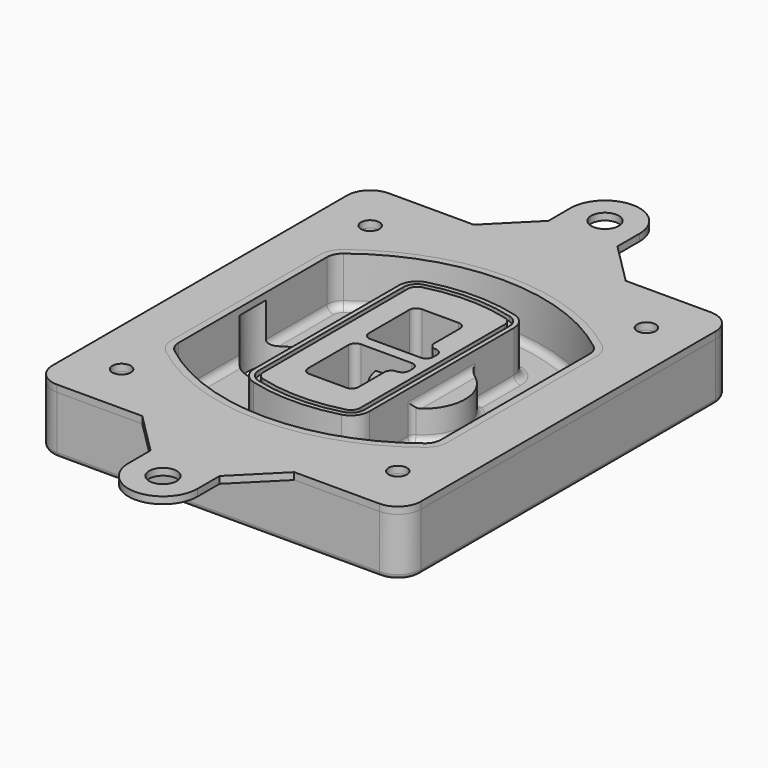
from build123d import *

# Parameters (mm, degrees)
F0_R      = 4
F1_DEPTH  = 25
F2_DEPTH  = 3
F3_DEPTH  = 18
F5_DEPTH  = 21
F6_DEPTH  = 2
F8_DEPTH  = 20
F9_DEPTH  = 16
F10_DEPTH = 25
F7_R      = 6
F7_R_2    = 4
F11_DEPTH = 6
F13_DEPTH = 9
F14_R     = 3
F15_R     = 2
F16_R     = 6
F16_R_2   = 4
F17_DEPTH = 3


# Not quite as in the source:
# - a feature names something its author has since deleted; it is built from what else it names


with BuildPart() as f1:
    # F0 (on Top) → F1 (new body)
    with BuildSketch(Plane.XY):
        with BuildLine():
            ThreePointArc((-80, -80), (-77.0710678119, -87.0710678119), (-70, -90))
            Line((-70, -90), (70, -90))
            ThreePointArc((70, -90), (77.0710678119, -87.0710678119), (80, -80))
            Line((80, -80), (80, 80))
            ThreePointArc((80, 80), (77.0710678119, 87.0710678119), (70, 90))
            Line((70, 90), (-70, 90))
            ThreePointArc((-70, 90), (-77.0710678119, 87.0710678119), (-80, 80))
            Line((-80, 80), (-80, -80))
        make_face()
        with Locations((-60, -67.5)):
            Circle(F0_R, mode=Mode.SUBTRACT)
        with Locations((60, -67.5)):
            Circle(F0_R, mode=Mode.SUBTRACT)
        with Locations((-60, 67.5)):
            Circle(F0_R, mode=Mode.SUBTRACT)
        with BuildLine():
            ThreePointArc((-64, 40.2934422872), (-62.5820384798, 46.4328484224), (-58.6153846154, 51.3286200352))
            ThreePointArc((-58.6153846154, 51.3286200352), (0, 71.5), (58.6153846154, 51.3286200352))
            ThreePointArc((58.6153846154, 51.3286200352), (62.5820384798, 46.4328484224), (64, 40.2934422872))
            Line((64, 40.2934422872), (64, -40.2934422872))
            ThreePointArc((64, -40.2934422872), (62.5820384798, -46.4328484224), (58.6153846154, -51.3286200352))
            ThreePointArc((58.6153846154, -51.3286200352), (0, -71.5), (-58.6153846154, -51.3286200352))
            ThreePointArc((-58.6153846154, -51.3286200352), (-62.5820384798, -46.4328484224), (-64, -40.2934422872))
            Line((-64, -40.2934422872), (-64, 40.2934422872))
        make_face(mode=Mode.SUBTRACT)
        with Locations((60, 67.5)):
            Circle(F0_R, mode=Mode.SUBTRACT)
        with BuildLine():
            ThreePointArc((58.6153846154, 51.3286200352), (0, 71.5), (-58.6153846154, 51.3286200352))
            ThreePointArc((-58.6153846154, 51.3286200352), (-62.5820384798, 46.4328484224), (-64, 40.2934422872))
            Line((-64, 40.2934422872), (-64, -40.2934422872))
            ThreePointArc((-64, -40.2934422872), (-62.5820384798, -46.4328484224), (-58.6153846154, -51.3286200352))
            ThreePointArc((-58.6153846154, -51.3286200352), (0, -71.5), (58.6153846154, -51.3286200352))
            ThreePointArc((58.6153846154, -51.3286200352), (62.5820384798, -46.4328484224), (64, -40.2934422872))
            Line((64, -40.2934422872), (64, 40.2934422872))
            ThreePointArc((64, 40.2934422872), (62.5820384798, 46.4328484224), (58.6153846154, 51.3286200352))
        make_face()
        with BuildLine():
            Line((-60, -40.2934422872), (-60, 40.2934422872))
            ThreePointArc((-60, 40.2934422872), (-58.9871703427, 44.6787323838), (-56.1538461538, 48.1757121072))
            ThreePointArc((-56.1538461538, 48.1757121072), (0, 67.5), (56.1538461538, 48.1757121072))
            ThreePointArc((56.1538461538, 48.1757121072), (58.9871703427, 44.6787323838), (60, 40.2934422872))
            Line((60, 40.2934422872), (60, -40.2934422872))
            ThreePointArc((60, -40.2934422872), (58.9871703427, -44.6787323838), (56.1538461538, -48.1757121072))
            ThreePointArc((56.1538461538, -48.1757121072), (0, -67.5), (-56.1538461538, -48.1757121072))
            ThreePointArc((-56.1538461538, -48.1757121072), (-58.9871703427, -44.6787323838), (-60, -40.2934422872))
        make_face(mode=Mode.SUBTRACT)
        with BuildLine():
            ThreePointArc((-56.1538461538, 48.1757121072), (-58.9871703427, 44.6787323838), (-60, 40.2934422872))
            Line((-60, 40.2934422872), (-60, -40.2934422872))
            ThreePointArc((-60, -40.2934422872), (-58.9871703427, -44.6787323838), (-56.1538461538, -48.1757121072))
            ThreePointArc((-56.1538461538, -48.1757121072), (0, -67.5), (56.1538461538, -48.1757121072))
            ThreePointArc((56.1538461538, -48.1757121072), (58.9871703427, -44.6787323838), (60, -40.2934422872))
            Line((60, -40.2934422872), (60, 40.2934422872))
            ThreePointArc((60, 40.2934422872), (58.9871703427, 44.6787323838), (56.1538461538, 48.1757121072))
            ThreePointArc((56.1538461538, 48.1757121072), (0, 67.5), (-56.1538461538, 48.1757121072))
        make_face()
        with BuildLine():
            ThreePointArc((54.3076923077, 45.8110311612), (56.2910192399, 43.3631453548), (57, 40.2934422872))
            Line((57, 40.2934422872), (57, -40.2934422872))
            ThreePointArc((57, -40.2934422872), (56.2910192399, -43.3631453548), (54.3076923077, -45.8110311612))
            ThreePointArc((54.3076923077, -45.8110311612), (0, -64.5), (-54.3076923077, -45.8110311612))
            ThreePointArc((-54.3076923077, -45.8110311612), (-56.2910192399, -43.3631453548), (-57, -40.2934422872))
            Line((-57, -40.2934422872), (-57, 40.2934422872))
            ThreePointArc((-57, 40.2934422872), (-56.2910192399, 43.3631453548), (-54.3076923077, 45.8110311612))
            ThreePointArc((-54.3076923077, 45.8110311612), (0, 64.5), (54.3076923077, 45.8110311612))
        make_face(mode=Mode.SUBTRACT)
        with BuildLine():
            Line((57, -40.2934422872), (57, 40.2934422872))
            ThreePointArc((57, 40.2934422872), (56.2910192399, 43.3631453548), (54.3076923077, 45.8110311612))
            ThreePointArc((54.3076923077, 45.8110311612), (0, 64.5), (-54.3076923077, 45.8110311612))
            ThreePointArc((-54.3076923077, 45.8110311612), (-56.2910192399, 43.3631453548), (-57, 40.2934422872))
            Line((-57, 40.2934422872), (-57, -40.2934422872))
            ThreePointArc((-57, -40.2934422872), (-56.2910192399, -43.3631453548), (-54.3076923077, -45.8110311612))
            ThreePointArc((-54.3076923077, -45.8110311612), (0, -64.5), (54.3076923077, -45.8110311612))
            ThreePointArc((54.3076923077, -45.8110311612), (56.2910192399, -43.3631453548), (57, -40.2934422872))
        make_face()
    extrude(amount=-F1_DEPTH)

    # F0 (on Top) → F2 (join)
    with BuildSketch(Plane.XY):
        with BuildLine():
            ThreePointArc((-56.1538461538, 48.1757121072), (-58.9871703427, 44.6787323838), (-60, 40.2934422872))
            Line((-60, 40.2934422872), (-60, -40.2934422872))
            ThreePointArc((-60, -40.2934422872), (-58.9871703427, -44.6787323838), (-56.1538461538, -48.1757121072))
            ThreePointArc((-56.1538461538, -48.1757121072), (0, -67.5), (56.1538461538, -48.1757121072))
            ThreePointArc((56.1538461538, -48.1757121072), (58.9871703427, -44.6787323838), (60, -40.2934422872))
            Line((60, -40.2934422872), (60, 40.2934422872))
            ThreePointArc((60, 40.2934422872), (58.9871703427, 44.6787323838), (56.1538461538, 48.1757121072))
            ThreePointArc((56.1538461538, 48.1757121072), (0, 67.5), (-56.1538461538, 48.1757121072))
        make_face()
        with BuildLine():
            ThreePointArc((54.3076923077, 45.8110311612), (56.2910192399, 43.3631453548), (57, 40.2934422872))
            Line((57, 40.2934422872), (57, -40.2934422872))
            ThreePointArc((57, -40.2934422872), (56.2910192399, -43.3631453548), (54.3076923077, -45.8110311612))
            ThreePointArc((54.3076923077, -45.8110311612), (0, -64.5), (-54.3076923077, -45.8110311612))
            ThreePointArc((-54.3076923077, -45.8110311612), (-56.2910192399, -43.3631453548), (-57, -40.2934422872))
            Line((-57, -40.2934422872), (-57, 40.2934422872))
            ThreePointArc((-57, 40.2934422872), (-56.2910192399, 43.3631453548), (-54.3076923077, 45.8110311612))
            ThreePointArc((-54.3076923077, 45.8110311612), (0, 64.5), (54.3076923077, 45.8110311612))
        make_face(mode=Mode.SUBTRACT)
    extrude(amount=F2_DEPTH)

    # F0 (on Top) → F3 (cut)
    with BuildSketch(Plane.XY):
        with BuildLine():
            Line((57, -40.2934422872), (57, 40.2934422872))
            ThreePointArc((57, 40.2934422872), (56.2910192399, 43.3631453548), (54.3076923077, 45.8110311612))
            ThreePointArc((54.3076923077, 45.8110311612), (0, 64.5), (-54.3076923077, 45.8110311612))
            ThreePointArc((-54.3076923077, 45.8110311612), (-56.2910192399, 43.3631453548), (-57, 40.2934422872))
            Line((-57, 40.2934422872), (-57, -40.2934422872))
            ThreePointArc((-57, -40.2934422872), (-56.2910192399, -43.3631453548), (-54.3076923077, -45.8110311612))
            ThreePointArc((-54.3076923077, -45.8110311612), (0, -64.5), (54.3076923077, -45.8110311612))
            ThreePointArc((54.3076923077, -45.8110311612), (56.2910192399, -43.3631453548), (57, -40.2934422872))
        make_face()
    extrude(amount=-F3_DEPTH, mode=Mode.SUBTRACT)

    # F4 (on face) → F5 (join, through all)
    with BuildSketch(Plane.XY.offset(3)):
        with BuildLine():
            ThreePointArc((-25, -39.2465276821), (-23.3511545998, -44.1109737193), (-19.0842911877, -46.9702398883))
            ThreePointArc((-19.0842911877, -46.9702398883), (0, -49.5), (19.0842911877, -46.9702398883))
            ThreePointArc((19.0842911877, -46.9702398883), (23.3511545998, -44.1109737193), (25, -39.2465276821))
            Line((25, -39.2465276821), (25, 39.2465276821))
            ThreePointArc((25, 39.2465276821), (23.3511545998, 44.1109737193), (19.0842911877, 46.9702398883))
            ThreePointArc((19.0842911877, 46.9702398883), (0, 49.5), (-19.0842911877, 46.9702398883))
            ThreePointArc((-19.0842911877, 46.9702398883), (-23.3511545998, 44.1109737193), (-25, 39.2465276821))
            Line((-25, 39.2465276821), (-25, -39.2465276821))
        make_face()
        with BuildLine():
            ThreePointArc((18.5632183908, 45.0393118368), (21.7633659499, 42.89486221), (23, 39.2465276821))
            Line((23, 39.2465276821), (23, -39.2465276821))
            ThreePointArc((23, -39.2465276821), (21.7633659499, -42.89486221), (18.5632183908, -45.0393118368))
            ThreePointArc((18.5632183908, -45.0393118368), (0, -47.5), (-18.5632183908, -45.0393118368))
            ThreePointArc((-18.5632183908, -45.0393118368), (-21.7633659499, -42.89486221), (-23, -39.2465276821))
            Line((-23, -39.2465276821), (-23, 39.2465276821))
            ThreePointArc((-23, 39.2465276821), (-21.7633659499, 42.89486221), (-18.5632183908, 45.0393118368))
            ThreePointArc((-18.5632183908, 45.0393118368), (0, 47.5), (18.5632183908, 45.0393118368))
        make_face(mode=Mode.SUBTRACT)
        with BuildLine():
            Line((23, -39.2465276821), (23, 39.2465276821))
            ThreePointArc((23, 39.2465276821), (21.7633659499, 42.89486221), (18.5632183908, 45.0393118368))
            ThreePointArc((18.5632183908, 45.0393118368), (0, 47.5), (-18.5632183908, 45.0393118368))
            ThreePointArc((-18.5632183908, 45.0393118368), (-21.7633659499, 42.89486221), (-23, 39.2465276821))
            Line((-23, 39.2465276821), (-23, -39.2465276821))
            ThreePointArc((-23, -39.2465276821), (-21.7633659499, -42.89486221), (-18.5632183908, -45.0393118368))
            ThreePointArc((-18.5632183908, -45.0393118368), (0, -47.5), (18.5632183908, -45.0393118368))
            ThreePointArc((18.5632183908, -45.0393118368), (21.7633659499, -42.89486221), (23, -39.2465276821))
        make_face()
        with BuildLine():
            ThreePointArc((18.0421455939, 43.1083837852), (20.1755772999, 41.6787507007), (21, 39.2465276821))
            Line((21, 39.2465276821), (21, -39.2465276821))
            ThreePointArc((21, -39.2465276821), (20.1755772999, -41.6787507007), (18.0421455939, -43.1083837852))
            ThreePointArc((18.0421455939, -43.1083837852), (0, -45.5), (-18.0421455939, -43.1083837852))
            ThreePointArc((-18.0421455939, -43.1083837852), (-20.1755772999, -41.6787507007), (-21, -39.2465276821))
            Line((-21, -39.2465276821), (-21, 39.2465276821))
            ThreePointArc((-21, 39.2465276821), (-20.1755772999, 41.6787507007), (-18.0421455939, 43.1083837852))
            ThreePointArc((-18.0421455939, 43.1083837852), (0, 45.5), (18.0421455939, 43.1083837852))
        make_face(mode=Mode.SUBTRACT)
        with BuildLine():
            Line((21, -39.2465276821), (21, 39.2465276821))
            ThreePointArc((21, 39.2465276821), (20.1755772999, 41.6787507007), (18.0421455939, 43.1083837852))
            ThreePointArc((18.0421455939, 43.1083837852), (0, 45.5), (-18.0421455939, 43.1083837852))
            ThreePointArc((-18.0421455939, 43.1083837852), (-20.1755772999, 41.6787507007), (-21, 39.2465276821))
            Line((-21, 39.2465276821), (-21, -39.2465276821))
            ThreePointArc((-21, -39.2465276821), (-20.1755772999, -41.6787507007), (-18.0421455939, -43.1083837852))
            ThreePointArc((-18.0421455939, -43.1083837852), (0, -45.5), (18.0421455939, -43.1083837852))
            ThreePointArc((18.0421455939, -43.1083837852), (20.1755772999, -41.6787507007), (21, -39.2465276821))
        make_face()
        with BuildLine():
            Line((-8, -2.5), (14, -2.5))
            ThreePointArc((14, -2.5), (16.1213203436, -3.3786796564), (17, -5.5))
            Line((17, -5.5), (17, -7.5))
            ThreePointArc((17, -7.5), (16.1213203436, -9.6213203436), (14, -10.5))
            ThreePointArc((14, -10.5), (11.8786796564, -11.3786796564), (11, -13.5))
            Line((11, -13.5), (11, -27.5))
            ThreePointArc((11, -27.5), (10.1213203436, -29.6213203436), (8, -30.5))
            Line((8, -30.5), (-8, -30.5))
            ThreePointArc((-8, -30.5), (-10.1213203436, -29.6213203436), (-11, -27.5))
            Line((-11, -27.5), (-11, -5.5))
            ThreePointArc((-11, -5.5), (-10.1213203436, -3.3786796564), (-8, -2.5))
        make_face(mode=Mode.SUBTRACT)
        with BuildLine():
            ThreePointArc((-8, 2.5), (-10.1213203436, 3.3786796564), (-11, 5.5))
            Line((-11, 5.5), (-11, 27.5))
            ThreePointArc((-11, 27.5), (-10.1213203436, 29.6213203436), (-8, 30.5))
            Line((-8, 30.5), (8, 30.5))
            ThreePointArc((8, 30.5), (10.1213203436, 29.6213203436), (11, 27.5))
            Line((11, 27.5), (11, 13.5))
            ThreePointArc((11, 13.5), (11.8786796564, 11.3786796564), (14, 10.5))
            ThreePointArc((14, 10.5), (16.1213203436, 9.6213203436), (17, 7.5))
            Line((17, 7.5), (17, 5.5))
            ThreePointArc((17, 5.5), (16.1213203436, 3.3786796564), (14, 2.5))
            Line((14, 2.5), (-8, 2.5))
        make_face(mode=Mode.SUBTRACT)
    extrude(amount=-F5_DEPTH)

    # F4 (on face) → F6 (cut)
    with BuildSketch(Plane.XY.offset(3)):
        with BuildLine():
            Line((23, -39.2465276821), (23, 39.2465276821))
            ThreePointArc((23, 39.2465276821), (21.7633659499, 42.89486221), (18.5632183908, 45.0393118368))
            ThreePointArc((18.5632183908, 45.0393118368), (0, 47.5), (-18.5632183908, 45.0393118368))
            ThreePointArc((-18.5632183908, 45.0393118368), (-21.7633659499, 42.89486221), (-23, 39.2465276821))
            Line((-23, 39.2465276821), (-23, -39.2465276821))
            ThreePointArc((-23, -39.2465276821), (-21.7633659499, -42.89486221), (-18.5632183908, -45.0393118368))
            ThreePointArc((-18.5632183908, -45.0393118368), (0, -47.5), (18.5632183908, -45.0393118368))
            ThreePointArc((18.5632183908, -45.0393118368), (21.7633659499, -42.89486221), (23, -39.2465276821))
        make_face()
        with BuildLine():
            ThreePointArc((18.0421455939, 43.1083837852), (20.1755772999, 41.6787507007), (21, 39.2465276821))
            Line((21, 39.2465276821), (21, -39.2465276821))
            ThreePointArc((21, -39.2465276821), (20.1755772999, -41.6787507007), (18.0421455939, -43.1083837852))
            ThreePointArc((18.0421455939, -43.1083837852), (0, -45.5), (-18.0421455939, -43.1083837852))
            ThreePointArc((-18.0421455939, -43.1083837852), (-20.1755772999, -41.6787507007), (-21, -39.2465276821))
            Line((-21, -39.2465276821), (-21, 39.2465276821))
            ThreePointArc((-21, 39.2465276821), (-20.1755772999, 41.6787507007), (-18.0421455939, 43.1083837852))
            ThreePointArc((-18.0421455939, 43.1083837852), (0, 45.5), (18.0421455939, 43.1083837852))
        make_face(mode=Mode.SUBTRACT)
    extrude(amount=-F6_DEPTH, mode=Mode.SUBTRACT)

    # F7 (on face) → F8 (join)
    with BuildSketch(Plane(origin=(0, 0, -25), x_dir=(1, 0, 0), z_dir=(0, 0, -1))):
        with BuildLine():
            ThreePointArc((3.28842436, 0), (16.7567035675, 13.4682792075), (30.224982775, 0))
            Line((30.224982775, 0), (35.224982775, 0))
            ThreePointArc((35.224982775, 0), (16.7567035675, 18.4682792075), (-1.71157564, 0))
            Line((-1.71157564, 0), (3.28842436, 0))
        make_face()
        with BuildLine():
            Line((3.28842436, 0), (30.224982775, 0))
            ThreePointArc((30.224982775, 0), (16.7567035675, 13.4682792075), (3.28842436, 0))
        make_face()
        with BuildLine():
            ThreePointArc((3.28842436, 0), (16.7567035675, -13.4682792075), (30.224982775, 0))
            Line((30.224982775, 0), (3.28842436, 0))
        make_face()
        with BuildLine():
            Line((35.224982775, 0), (30.224982775, 0))
            ThreePointArc((30.224982775, 0), (16.7567035675, -13.4682792075), (3.28842436, 0))
            Line((3.28842436, 0), (-1.71157564, 0))
            ThreePointArc((-1.71157564, 0), (16.7567035675, -18.4682792075), (35.224982775, 0))
        make_face()
    extrude(amount=-F8_DEPTH)

    # F7 (on face) → F9 (cut)
    with BuildSketch(Plane(origin=(0, 0, -25), x_dir=(1, 0, 0), z_dir=(0, 0, -1))):
        with BuildLine():
            Line((3.28842436, 0), (30.224982775, 0))
            ThreePointArc((30.224982775, 0), (16.7567035675, 13.4682792075), (3.28842436, 0))
        make_face()
        with BuildLine():
            ThreePointArc((3.28842436, 0), (16.7567035675, -13.4682792075), (30.224982775, 0))
            Line((30.224982775, 0), (3.28842436, 0))
        make_face()
    extrude(amount=-F9_DEPTH, mode=Mode.SUBTRACT)

    # F7 (on face) → F10 (cut)
    with BuildSketch(Plane(origin=(0, 0, -25), x_dir=(1, 0, 0), z_dir=(0, 0, -1))):
        with BuildLine():
            Line((-59.0318229325, 0), (-32.0952645175, 0))
            ThreePointArc((-32.0952645175, 0), (-45.563543725, 13.4682792075), (-59.0318229325, 0))
        make_face()
        with BuildLine():
            ThreePointArc((-59.0318229325, 0), (-45.563543725, -13.4682792075), (-32.0952645175, 0))
            Line((-32.0952645175, 0), (-59.0318229325, 0))
        make_face()
    extrude(amount=-F10_DEPTH, mode=Mode.SUBTRACT)

    # F7 (on face) → F11 (cut)
    with BuildSketch(Plane(origin=(0, 0, -25), x_dir=(1, 0, 0), z_dir=(0, 0, -1))):
        with Locations((60, -67.5)):
            Circle(F7_R)
        with Locations((60, -67.5)):
            Circle(F7_R_2, mode=Mode.SUBTRACT)
        with Locations((-60, -67.5)):
            Circle(F7_R)
        with Locations((-60, -67.5)):
            Circle(F7_R_2, mode=Mode.SUBTRACT)
        with Locations((-60, 67.5)):
            Circle(F7_R)
        with Locations((-60, 67.5)):
            Circle(F7_R_2, mode=Mode.SUBTRACT)
        with Locations((60, 67.5)):
            Circle(F7_R)
        with Locations((60, 67.5)):
            Circle(F7_R_2, mode=Mode.SUBTRACT)
    extrude(amount=-F11_DEPTH, mode=Mode.SUBTRACT)

    # F12 (on face) → F13 (cut, through all)
    with BuildSketch(Plane(origin=(0, 0, -9), x_dir=(1, 0, 0), z_dir=(0, 0, -1))):
        with BuildLine():
            Line((11, 13.5), (11, 17.5481537753))
            ThreePointArc((11, 17.5481537753), (2.5696536419, 11.8239143813), (-1.5415842455, 2.5))
            Line((-1.5415842455, 2.5), (3.5224848595, 2.5))
            ThreePointArc((3.5224848595, 2.5), (6.1857188154, 8.3455872281), (11.2536447004, 12.2927168648))
            ThreePointArc((11.2536447004, 12.2927168648), (11.0640958889, 12.8831798879), (11, 13.5))
        make_face()
        with BuildLine():
            ThreePointArc((11.2536447004, -12.2927168648), (6.1857188154, -8.3455872281), (3.5224848595, -2.5))
            Line((3.5224848595, -2.5), (-1.5415842455, -2.5))
            ThreePointArc((-1.5415842455, -2.5), (2.5696536419, -11.8239143813), (11, -17.5481537753))
            Line((11, -17.5481537753), (11, -13.5))
            ThreePointArc((11, -13.5), (11.0640958889, -12.8831798879), (11.2536447004, -12.2927168648))
        make_face()
        with BuildLine():
            ThreePointArc((11.2536447004, 12.2927168648), (6.1857188154, 8.3455872281), (3.5224848595, 2.5))
            Line((3.5224848595, 2.5), (14, 2.5))
            ThreePointArc((14, 2.5), (16.1213203436, 3.3786796564), (17, 5.5))
            Line((17, 5.5), (17, 7.5))
            ThreePointArc((17, 7.5), (16.1213203436, 9.6213203436), (14, 10.5))
            ThreePointArc((14, 10.5), (12.3601599782, 10.9878446101), (11.2536447004, 12.2927168648))
        make_face()
        with BuildLine():
            Line((14, -2.5), (3.5224848595, -2.5))
            ThreePointArc((3.5224848595, -2.5), (6.1857188154, -8.3455872281), (11.2536447004, -12.2927168648))
            ThreePointArc((11.2536447004, -12.2927168648), (12.3601599782, -10.9878446101), (14, -10.5))
            ThreePointArc((14, -10.5), (16.1213203436, -9.6213203436), (17, -7.5))
            Line((17, -7.5), (17, -5.5))
            ThreePointArc((17, -5.5), (16.1213203436, -3.3786796564), (14, -2.5))
        make_face()
    extrude(amount=F13_DEPTH, mode=Mode.SUBTRACT)

    # F14
    f14_edges = [f1.edges().sort_by_distance(p)[0] for p in [
        (-57, -23.703476, -18),
        (-57, 23.703476, -18),
        (25, 0, -5),
        (25, 16.526506, -11.5),
        (25, -16.526506, -11.5),
        (25, -27.886517, -18),
        (35.224983, 0, -18),
    ]]
    fillet(f14_edges, radius=F14_R)

    # F15
    f15_edges = [f1.edges().sort_by_distance(p)[0] for p in [
        (0, -90, -25),
    ]]
    fillet(f15_edges, radius=F15_R)


with BuildPart() as f17:
    # F16 (on face) → F17 (new body, through all)
    with BuildSketch(Plane.XY):
        with BuildLine():
            Line((-15, 108), (-33, 90))
            Line((-33, 90), (33, 90))
            Line((33, 90), (15, 108))
            Line((15, 108), (15, 120))
            ThreePointArc((15, 120), (0, 135), (-15, 120))
            Line((-15, 120), (-15, 108))
        make_face()
        with Locations((0, 120)):
            Circle(F16_R, mode=Mode.SUBTRACT)
        with BuildLine():
            Line((33, -90), (-33, -90))
            Line((-33, -90), (-15, -108))
            Line((-15, -108), (-15, -120))
            ThreePointArc((-15, -120), (0, -135), (15, -120))
            Line((15, -120), (15, -108))
            Line((15, -108), (33, -90))
        make_face()
        with Locations((0, -120)):
            Circle(F16_R, mode=Mode.SUBTRACT)
        with BuildLine():
            Line((33, 90), (-33, 90))
            Line((-33, 90), (-70, 90))
            ThreePointArc((-70, 90), (-77.0710678119, 87.0710678119), (-80, 80))
            Line((-80, 80), (-80, -80))
            ThreePointArc((-80, -80), (-77.0710678119, -87.0710678119), (-70, -90))
            Line((-70, -90), (-33, -90))
            Line((-33, -90), (33, -90))
            Line((33, -90), (70, -90))
            ThreePointArc((70, -90), (77.0710678119, -87.0710678119), (80, -80))
            Line((80, -80), (80, 80))
            ThreePointArc((80, 80), (77.0710678119, 87.0710678119), (70, 90))
            Line((70, 90), (33, 90))
        make_face()
        with Locations((-60, -67.5)):
            Circle(F16_R_2, mode=Mode.SUBTRACT)
        with Locations((60, -67.5)):
            Circle(F16_R_2, mode=Mode.SUBTRACT)
        with Locations((-60, 67.5)):
            Circle(F16_R_2, mode=Mode.SUBTRACT)
        with BuildLine():
            ThreePointArc((-60, 40.2934422872), (-58.9871703427, 44.6787323838), (-56.1538461538, 48.1757121072))
            ThreePointArc((-56.1538461538, 48.1757121072), (0, 67.5), (56.1538461538, 48.1757121072))
            ThreePointArc((56.1538461538, 48.1757121072), (58.9871703427, 44.6787323838), (60, 40.2934422872))
            Line((60, 40.2934422872), (60, -40.2934422872))
            ThreePointArc((60, -40.2934422872), (58.9871703427, -44.6787323838), (56.1538461538, -48.1757121072))
            ThreePointArc((56.1538461538, -48.1757121072), (0, -67.5), (-56.1538461538, -48.1757121072))
            ThreePointArc((-56.1538461538, -48.1757121072), (-58.9871703427, -44.6787323838), (-60, -40.2934422872))
            Line((-60, -40.2934422872), (-60, 40.2934422872))
        make_face(mode=Mode.SUBTRACT)
        with Locations((60, 67.5)):
            Circle(F16_R_2, mode=Mode.SUBTRACT)
    extrude(amount=F17_DEPTH)


solid = Compound([f1.part, f17.part])
